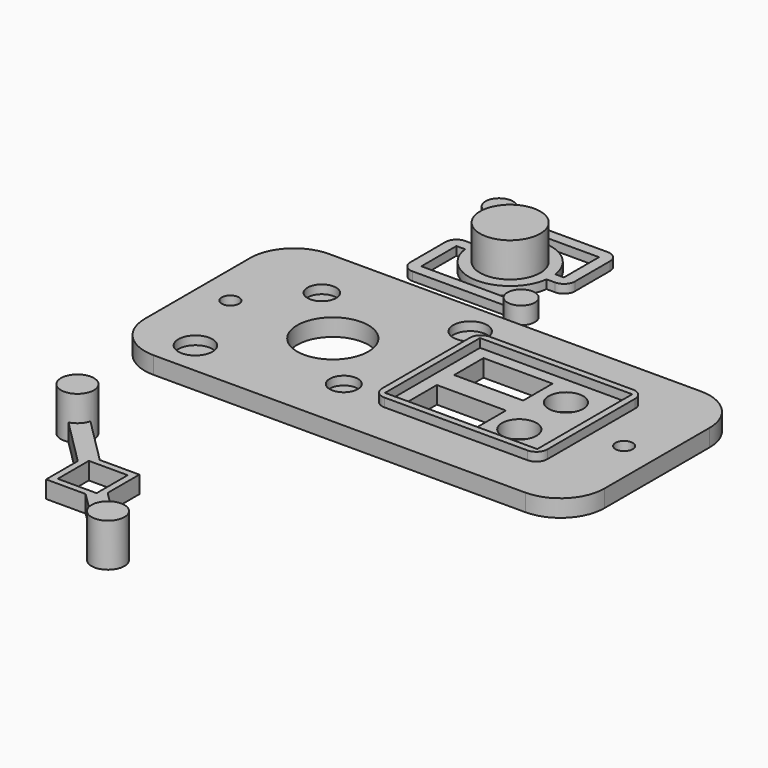
from build123d import *

# Parameters (mm, degrees)
F0_W      = 106.426
F0_H      = 50.8
F0_R      = 3.937
F0_R_2    = 3.2593015929
F0_R_3    = 2
F0_R_4    = 8.255
F0_R_5    = 3.302
F0_W_2    = 38.25
F0_H_2    = 30.5
F0_W_3    = 35.25
F0_H_3    = 27.5
F0_W_4    = 16
F0_H_4    = 8.5
F0_R_6    = 4
F1_DEPTH  = 4
F2_R      = 10.16
F3_DEPTH  = 6
F4_R      = 6.985
F4_W      = 1.27
F4_H      = 10.16
F4_H_2    = 1.27
F4_W_2    = 3
F4_H_3    = 4
F5_DEPTH  = 2
F6_DEPTH  = 10
F7_R      = 2.54
F8_DEPTH  = 4
F9_DEPTH  = 4
F10_START = 2
F10_DEPTH = 2
F11_W     = 9
F11_H     = 9
F12_DEPTH = 4
F13_R     = 2.54
F14_DEPTH = 10


# Not quite as in the source:
# - a feature names something its author has since deleted; it is built from what else it names


with BuildPart() as f1:
    # F0 (on Top) → F1 (new body)
    with BuildSketch(Plane.XY):
        with Locations((-3.608, -5.1e-06)):
            Rectangle(F0_W, F0_H)
        with Locations((-43.1534, -17.6784)):
            Circle(F0_R, mode=Mode.SUBTRACT)
        with Locations((-12.775, -12.7)):
            Circle(F0_R_2, mode=Mode.SUBTRACT)
        with Locations((-49.201, 0.0028)):
            Circle(F0_R_3, mode=Mode.SUBTRACT)
        with Locations((-25.475, 0)):
            Circle(F0_R_4, mode=Mode.SUBTRACT)
        with Locations((-38.175, 12.7)):
            Circle(F0_R_5, mode=Mode.SUBTRACT)
        with Locations((-7.7966, 17.6784)):
            Circle(F0_R, mode=Mode.SUBTRACT)
        with Locations((15.24, 0)):
            Rectangle(F0_W_2, F0_H_2, mode=Mode.SUBTRACT)
        with Locations((41.985, 0.0028)):
            Circle(F0_R_3, mode=Mode.SUBTRACT)
        with Locations((15.24, 0)):
            Rectangle(F0_W_2, F0_H_2)
        with Locations((15.24, 0)):
            Rectangle(F0_W_3, F0_H_3, mode=Mode.SUBTRACT)
        with Locations((15.24, 0)):
            Rectangle(F0_W_3, F0_H_3)
        with Locations((8.615, -6.75)):
            Rectangle(F0_W_4, F0_H_4, mode=Mode.SUBTRACT)
        with Locations((23.115, -6.75)):
            Circle(F0_R_6, mode=Mode.SUBTRACT)
        with Locations((8.615, 6.75)):
            Rectangle(F0_W_4, F0_H_4, mode=Mode.SUBTRACT)
        with Locations((23.115, 6.75)):
            Circle(F0_R_6, mode=Mode.SUBTRACT)
        with Locations((-38.175, 12.7)):
            Circle(F0_R_5)
        with Locations((-12.775, -12.7)):
            Circle(F0_R_2)
        with Locations((-7.7966, 17.6784)):
            Circle(F0_R)
        with Locations((-43.1534, -17.6784)):
            Circle(F0_R)
    extrude(amount=F1_DEPTH)

    # F2
    f2_edges = [f1.edges().sort_by_distance(p)[0] for p in [
        (-56.821, -25.400005, 2),
        (-56.821, 25.399995, 2),
        (49.605, 25.399995, 2),
        (49.605, -25.400005, 2),
    ]]
    fillet(f2_edges, radius=F2_R)

    # F0 (on Top) → F3 (join)
    with BuildSketch(Plane.XY):
        with Locations((15.24, 0)):
            Rectangle(F0_W_2, F0_H_2)
        with Locations((15.24, 0)):
            Rectangle(F0_W_3, F0_H_3, mode=Mode.SUBTRACT)
    extrude(amount=F3_DEPTH)

    # F0 (on Top) → F10 (cut)
    with BuildSketch(Plane.XY.offset(F10_START)):
        with Locations((-38.175, 12.7)):
            Circle(F0_R_5)
        with Locations((-12.775, -12.7)):
            Circle(F0_R_2)
        with Locations((-7.7966, 17.6784)):
            Circle(F0_R)
        with Locations((-43.1534, -17.6784)):
            Circle(F0_R)
    extrude(amount=F10_DEPTH, mode=Mode.SUBTRACT)

    # F13
    f13_edges = [f1.edges().sort_by_distance(p)[0] for p in [
        (-3.885, 15.25, 5),
        (34.365, 15.25, 5),
        (34.365, -15.25, 5),
        (-3.885, -15.25, 5),
    ]]
    fillet(f13_edges, radius=F13_R)


with BuildPart() as f5:
    # F4 (on Top) → F5 (new body)
    with BuildSketch(Plane.XY):
        with BuildLine():
            Line((-13.3349857867, 47.7519830668), (-12.1500321321, 47.7519830668))
            ThreePointArc((-12.1500321321, 47.7519830668), (-21.5899857867, 56.0069830668), (-31.0299394412, 47.7519830668))
            Line((-31.0299394412, 47.7519830668), (-29.8449857867, 47.7519830668))
            Line((-29.8449857867, 47.7519830668), (-29.8449857867, 45.2119830668))
            Line((-29.8449857867, 45.2119830668), (-31.0299394412, 45.2119830668))
            ThreePointArc((-31.0299394412, 45.2119830668), (-21.5899857867, 36.9569830668), (-12.1500321321, 45.2119830668))
            Line((-12.1500321321, 45.2119830668), (-13.3349857867, 45.2119830668))
            Line((-13.3349857867, 45.2119830668), (-13.3349857867, 47.7519830668))
        make_face()
        with Locations((-21.5899857867, 46.4819830668)):
            Circle(F4_R, mode=Mode.SUBTRACT)
        with BuildLine():
            ThreePointArc((-5.7149857867, 33.7819830668), (-8.241302668, 36.8900106104), (-11.799921353, 35.0519830668))
            Line((-11.799921353, 35.0519830668), (-7.6199857867, 35.0519830668))
            Line((-7.6199857867, 35.0519830668), (-7.6199857867, 32.5119830668))
            Line((-7.6199857867, 32.5119830668), (-11.799921353, 32.5119830668))
            ThreePointArc((-11.799921353, 32.5119830668), (-8.241302668, 30.6739555232), (-5.7149857867, 33.7819830668))
        make_face()
        with BuildLine():
            ThreePointArc((-31.3800502204, 60.4519830668), (-37.4649857867, 59.1819830668), (-31.3800502204, 57.9119830668))
            Line((-31.3800502204, 57.9119830668), (-34.2899857867, 57.9119830668))
            Line((-34.2899857867, 57.9119830668), (-34.2899857867, 59.1819830668))
            Line((-34.2899857867, 59.1819830668), (-34.2899857867, 60.4519830668))
            Line((-34.2899857867, 60.4519830668), (-31.3800502204, 60.4519830668))
        make_face()
        with BuildLine():
            ThreePointArc((-31.1149857867, 59.1819830668), (-31.1819582431, 59.8306661855), (-31.3800502204, 60.4519830668))
            Line((-31.3800502204, 60.4519830668), (-34.2899857867, 60.4519830668))
            Line((-34.2899857867, 60.4519830668), (-34.2899857867, 59.1819830668))
            Line((-34.2899857867, 59.1819830668), (-31.1149857867, 59.1819830668))
        make_face()
        with BuildLine():
            Line((-34.2899857867, 57.9119830668), (-31.3800502204, 57.9119830668))
            ThreePointArc((-31.3800502204, 57.9119830668), (-31.1819582431, 58.5332999481), (-31.1149857867, 59.1819830668))
            Line((-31.1149857867, 59.1819830668), (-34.2899857867, 59.1819830668))
            Line((-34.2899857867, 59.1819830668), (-34.2899857867, 57.9119830668))
        make_face()
        with BuildLine():
            Line((-31.3800502204, 57.9119830668), (-10.1599857867, 57.9119830668))
            Line((-10.1599857867, 57.9119830668), (-10.1599857867, 59.1819830668))
            Line((-10.1599857867, 59.1819830668), (-31.1149857867, 59.1819830668))
            ThreePointArc((-31.1149857867, 59.1819830668), (-31.1819582431, 58.5332999481), (-31.3800502204, 57.9119830668))
        make_face()
        with BuildLine():
            Line((-31.1149857867, 59.1819830668), (-10.1599857867, 59.1819830668))
            Line((-10.1599857867, 59.1819830668), (-10.1599857867, 60.4519830668))
            Line((-10.1599857867, 60.4519830668), (-31.3800502204, 60.4519830668))
            ThreePointArc((-31.3800502204, 60.4519830668), (-31.1819582431, 59.8306661855), (-31.1149857867, 59.1819830668))
        make_face()
        Polygon((-8.8899857867, 57.9119830668), (-8.8899857867, 47.7519830668), (-7.6199857867, 47.7519830668), (-7.6199857867, 60.4519830668), (-8.8899857867, 60.4519830668), (-8.8899857867, 59.1819830668), align=None)
        with Locations((-9.5249857867, 52.8319830668)):
            Rectangle(F4_W, F4_H)
        with Locations((-9.5249857867, 58.5469830668)):
            Rectangle(F4_W, F4_H_2)
        with Locations((-9.5249857867, 59.8169830668)):
            Rectangle(F4_W, F4_H_2)
        Polygon((-8.8899857867, 46.4819830668), (-10.1599857867, 46.4819830668), (-10.1599857867, 45.2119830668), (-7.6199857867, 45.2119830668), (-7.6199857867, 47.7519830668), (-8.8899857867, 47.7519830668), align=None)
        with Locations((-9.5249857867, 47.1169830668)):
            Rectangle(F4_W, F4_H_2)
        with BuildLine():
            ThreePointArc((-12.1500321321, 47.7519830668), (-12.0862711561, 47.1184052696), (-12.0649857867, 46.4819830668))
            Line((-12.0649857867, 46.4819830668), (-10.1599857867, 46.4819830668))
            Line((-10.1599857867, 46.4819830668), (-10.1599857867, 47.7519830668))
            Line((-10.1599857867, 47.7519830668), (-12.1500321321, 47.7519830668))
        make_face()
        with BuildLine():
            Line((-10.1599857867, 46.4819830668), (-12.0649857867, 46.4819830668))
            ThreePointArc((-12.0649857867, 46.4819830668), (-12.0862711561, 45.845560864), (-12.1500321321, 45.2119830668))
            Line((-12.1500321321, 45.2119830668), (-10.1599857867, 45.2119830668))
            Line((-10.1599857867, 45.2119830668), (-10.1599857867, 46.4819830668))
        make_face()
        with BuildLine():
            ThreePointArc((-12.1500321321, 45.2119830668), (-12.0862711561, 45.845560864), (-12.0649857867, 46.4819830668))
            ThreePointArc((-12.0649857867, 46.4819830668), (-12.0862711561, 47.1184052696), (-12.1500321321, 47.7519830668))
            Line((-12.1500321321, 47.7519830668), (-13.3349857867, 47.7519830668))
            Line((-13.3349857867, 47.7519830668), (-13.3349857867, 45.2119830668))
            Line((-13.3349857867, 45.2119830668), (-12.1500321321, 45.2119830668))
        make_face()
        with BuildLine():
            ThreePointArc((-31.1149857867, 46.4819830668), (-31.0937004173, 47.1184052696), (-31.0299394412, 47.7519830668))
            Line((-31.0299394412, 47.7519830668), (-33.0199857867, 47.7519830668))
            Line((-33.0199857867, 47.7519830668), (-33.0199857867, 46.4819830668))
            Line((-33.0199857867, 46.4819830668), (-31.1149857867, 46.4819830668))
        make_face()
        with BuildLine():
            Line((-33.0199857867, 45.2119830668), (-31.0299394412, 45.2119830668))
            ThreePointArc((-31.0299394412, 45.2119830668), (-31.0937004173, 45.845560864), (-31.1149857867, 46.4819830668))
            Line((-31.1149857867, 46.4819830668), (-33.0199857867, 46.4819830668))
            Line((-33.0199857867, 46.4819830668), (-33.0199857867, 45.2119830668))
        make_face()
        with BuildLine():
            Line((-29.8449857867, 47.7519830668), (-31.0299394412, 47.7519830668))
            ThreePointArc((-31.0299394412, 47.7519830668), (-31.0937004173, 47.1184052696), (-31.1149857867, 46.4819830668))
            ThreePointArc((-31.1149857867, 46.4819830668), (-31.0937004173, 45.845560864), (-31.0299394412, 45.2119830668))
            Line((-31.0299394412, 45.2119830668), (-29.8449857867, 45.2119830668))
            Line((-29.8449857867, 45.2119830668), (-29.8449857867, 47.7519830668))
        make_face()
        Polygon((-33.0199857867, 46.4819830668), (-33.0199857867, 47.7519830668), (-35.5599857867, 47.7519830668), (-35.5599857867, 45.2119830668), (-34.2899857867, 45.2119830668), (-34.2899857867, 46.4819830668), align=None)
        with Locations((-33.6549857867, 45.8469830668)):
            Rectangle(F4_W, F4_H_2)
        with Locations((-34.9249857867, 40.1319830668)):
            Rectangle(F4_W, F4_H)
        with Locations((-33.6549857867, 40.1319830668)):
            Rectangle(F4_W, F4_H)
        Polygon((-34.2899857867, 33.7819830668), (-34.2899857867, 35.0519830668), (-35.5599857867, 35.0519830668), (-35.5599857867, 32.5119830668), (-33.0199857867, 32.5119830668), (-33.0199857867, 33.7819830668), align=None)
        with Locations((-33.6549857867, 34.4169830668)):
            Rectangle(F4_W, F4_H_2)
        with BuildLine():
            Line((-11.799921353, 35.0519830668), (-33.0199857867, 35.0519830668))
            Line((-33.0199857867, 35.0519830668), (-33.0199857867, 33.7819830668))
            Line((-33.0199857867, 33.7819830668), (-12.0649857867, 33.7819830668))
            ThreePointArc((-12.0649857867, 33.7819830668), (-11.9980133302, 34.4306661855), (-11.799921353, 35.0519830668))
        make_face()
        with BuildLine():
            Line((-12.0649857867, 33.7819830668), (-33.0199857867, 33.7819830668))
            Line((-33.0199857867, 33.7819830668), (-33.0199857867, 32.5119830668))
            Line((-33.0199857867, 32.5119830668), (-11.799921353, 32.5119830668))
            ThreePointArc((-11.799921353, 32.5119830668), (-11.9980133302, 33.1332999481), (-12.0649857867, 33.7819830668))
        make_face()
        with BuildLine():
            Line((-7.6199857867, 35.0519830668), (-11.799921353, 35.0519830668))
            ThreePointArc((-11.799921353, 35.0519830668), (-11.9980133302, 34.4306661855), (-12.0649857867, 33.7819830668))
            ThreePointArc((-12.0649857867, 33.7819830668), (-11.9980133302, 33.1332999481), (-11.799921353, 32.5119830668))
            Line((-11.799921353, 32.5119830668), (-7.6199857867, 32.5119830668))
            Line((-7.6199857867, 32.5119830668), (-7.6199857867, 35.0519830668))
        make_face()
        with Locations((-21.5899857867, 46.4819830668)):
            Circle(F4_R)
        with Locations((-21.5899857867, 46.4819830668)):
            Rectangle(F4_W_2, F4_H_3, mode=Mode.SUBTRACT)
        with Locations((-21.5899857867, 46.4819830668)):
            Rectangle(F4_W_2, F4_H_3)
    extrude(amount=F5_DEPTH)

    # F4 (on Top) → F6 (join)
    with BuildSketch(Plane.XY):
        with Locations((-21.5899857867, 46.4819830668)):
            Circle(F4_R)
        with Locations((-21.5899857867, 46.4819830668)):
            Rectangle(F4_W_2, F4_H_3, mode=Mode.SUBTRACT)
        with Locations((-21.5899857867, 46.4819830668)):
            Rectangle(F4_W_2, F4_H_3)
    extrude(amount=F6_DEPTH)

    # F7
    f7_edges = [f5.edges().sort_by_distance(p)[0] for p in [
        (-7.619986, 60.451983, 1),
        (-7.619986, 45.211983, 1),
        (-35.559986, 32.511983, 1),
        (-35.559986, 47.751983, 1),
    ]]
    fillet(f7_edges, radius=F7_R)

    # F4 (on Top) → F8 (cut)
    with BuildSketch(Plane.XY):
        with Locations((-21.5899857867, 46.4819830668)):
            Rectangle(F4_W_2, F4_H_3)
    extrude(amount=F8_DEPTH, mode=Mode.SUBTRACT)

    # F4 (on Top) → F9 (join)
    with BuildSketch(Plane.XY):
        with BuildLine():
            ThreePointArc((-31.3800502204, 60.4519830668), (-37.4649857867, 59.1819830668), (-31.3800502204, 57.9119830668))
            Line((-31.3800502204, 57.9119830668), (-34.2899857867, 57.9119830668))
            Line((-34.2899857867, 57.9119830668), (-34.2899857867, 59.1819830668))
            Line((-34.2899857867, 59.1819830668), (-34.2899857867, 60.4519830668))
            Line((-34.2899857867, 60.4519830668), (-31.3800502204, 60.4519830668))
        make_face()
        with BuildLine():
            ThreePointArc((-31.1149857867, 59.1819830668), (-31.1819582431, 59.8306661855), (-31.3800502204, 60.4519830668))
            Line((-31.3800502204, 60.4519830668), (-34.2899857867, 60.4519830668))
            Line((-34.2899857867, 60.4519830668), (-34.2899857867, 59.1819830668))
            Line((-34.2899857867, 59.1819830668), (-31.1149857867, 59.1819830668))
        make_face()
        with BuildLine():
            Line((-34.2899857867, 57.9119830668), (-31.3800502204, 57.9119830668))
            ThreePointArc((-31.3800502204, 57.9119830668), (-31.1819582431, 58.5332999481), (-31.1149857867, 59.1819830668))
            Line((-31.1149857867, 59.1819830668), (-34.2899857867, 59.1819830668))
            Line((-34.2899857867, 59.1819830668), (-34.2899857867, 57.9119830668))
        make_face()
        with BuildLine():
            ThreePointArc((-5.7149857867, 33.7819830668), (-8.241302668, 36.8900106104), (-11.799921353, 35.0519830668))
            Line((-11.799921353, 35.0519830668), (-7.6199857867, 35.0519830668))
            Line((-7.6199857867, 35.0519830668), (-7.6199857867, 32.5119830668))
            Line((-7.6199857867, 32.5119830668), (-11.799921353, 32.5119830668))
            ThreePointArc((-11.799921353, 32.5119830668), (-8.241302668, 30.6739555232), (-5.7149857867, 33.7819830668))
        make_face()
        with BuildLine():
            Line((-7.6199857867, 35.0519830668), (-11.799921353, 35.0519830668))
            ThreePointArc((-11.799921353, 35.0519830668), (-11.9980133302, 34.4306661855), (-12.0649857867, 33.7819830668))
            ThreePointArc((-12.0649857867, 33.7819830668), (-11.9980133302, 33.1332999481), (-11.799921353, 32.5119830668))
            Line((-11.799921353, 32.5119830668), (-7.6199857867, 32.5119830668))
            Line((-7.6199857867, 32.5119830668), (-7.6199857867, 35.0519830668))
        make_face()
    extrude(amount=F9_DEPTH)


with BuildPart() as f12:
    # F11 (on Top) → F12 (new body)
    with BuildSketch(Plane.XY):
        with BuildLine():
            ThreePointArc((-42.2705026911, -55.5329295336), (-41.2924403918, -55.152540039), (-40.4552561211, -54.5197489789))
            ThreePointArc((-40.4552561211, -54.5197489789), (-39.822465061, -53.6825647082), (-39.4420755664, -52.7045024089))
            ThreePointArc((-39.4420755664, -52.7045024089), (-39.36510578, -52.2680799524), (-39.3393329574, -51.8256721426))
            ThreePointArc((-39.3393329574, -51.8256721426), (-46.1380152184, -49.4626490063), (-42.2705026911, -55.5329295336))
        make_face()
        with BuildLine():
            Line((-40.4552561211, -54.5197489789), (-31.475, -63.5000051))
            Line((-31.475, -63.5000051), (-28.6465728753, -63.5000051))
            Line((-28.6465728753, -63.5000051), (-39.4420755664, -52.7045024089))
            ThreePointArc((-39.4420755664, -52.7045024089), (-39.822465061, -53.6825647082), (-40.4552561211, -54.5197489789))
        make_face()
        with BuildLine():
            Line((-31.475, -66.3284322247), (-31.475, -63.5000051))
            Line((-31.475, -63.5000051), (-40.4552561211, -54.5197489789))
            ThreePointArc((-40.4552561211, -54.5197489789), (-41.2924403918, -55.152540039), (-42.2705026911, -55.5329295336))
            Line((-42.2705026911, -55.5329295336), (-31.475, -66.3284322247))
        make_face()
        Polygon((-28.6465728753, -63.5000051), (-31.475, -63.5000051), (-31.475, -66.3284322247), (-31.475, -75.5000051), (-22.3034271247, -75.5000051), (-19.475, -75.5000051), (-19.475, -72.6715779753), (-19.475, -63.5000051), align=None)
        with Locations((-25.475, -69.5000051)):
            Rectangle(F11_W, F11_H, mode=Mode.SUBTRACT)
        with BuildLine():
            Line((-8.6794973089, -83.4670806664), (-19.475, -72.6715779753))
            Line((-19.475, -72.6715779753), (-19.475, -75.5000051))
            Line((-19.475, -75.5000051), (-10.4947438789, -84.4802612211))
            ThreePointArc((-10.4947438789, -84.4802612211), (-9.6575596082, -83.847470161), (-8.6794973089, -83.4670806664))
        make_face()
        with BuildLine():
            Line((-19.475, -75.5000051), (-22.3034271247, -75.5000051))
            Line((-22.3034271247, -75.5000051), (-11.5079244336, -86.2955077911))
            ThreePointArc((-11.5079244336, -86.2955077911), (-11.127534939, -85.3174454918), (-10.4947438789, -84.4802612211))
            Line((-10.4947438789, -84.4802612211), (-19.475, -75.5000051))
        make_face()
        with BuildLine():
            ThreePointArc((-3.9906670426, -87.1743380574), (-5.4376439063, -84.1856557964), (-8.6794973089, -83.4670806664))
            ThreePointArc((-8.6794973089, -83.4670806664), (-9.6575596082, -83.847470161), (-10.4947438789, -84.4802612211))
            ThreePointArc((-10.4947438789, -84.4802612211), (-11.127534939, -85.3174454918), (-11.5079244336, -86.2955077911))
            ThreePointArc((-11.5079244336, -86.2955077911), (-8.2430748524, -90.9585652347), (-3.9906670426, -87.1743380574))
        make_face()
    extrude(amount=F12_DEPTH)

    # F11 (on Top) → F14 (join)
    with BuildSketch(Plane.XY):
        with BuildLine():
            ThreePointArc((-42.2705026911, -55.5329295336), (-41.2924403918, -55.152540039), (-40.4552561211, -54.5197489789))
            ThreePointArc((-40.4552561211, -54.5197489789), (-39.822465061, -53.6825647082), (-39.4420755664, -52.7045024089))
            ThreePointArc((-39.4420755664, -52.7045024089), (-39.36510578, -52.2680799524), (-39.3393329574, -51.8256721426))
            ThreePointArc((-39.3393329574, -51.8256721426), (-46.1380152184, -49.4626490063), (-42.2705026911, -55.5329295336))
        make_face()
        with BuildLine():
            ThreePointArc((-3.9906670426, -87.1743380574), (-5.4376439063, -84.1856557964), (-8.6794973089, -83.4670806664))
            ThreePointArc((-8.6794973089, -83.4670806664), (-9.6575596082, -83.847470161), (-10.4947438789, -84.4802612211))
            ThreePointArc((-10.4947438789, -84.4802612211), (-11.127534939, -85.3174454918), (-11.5079244336, -86.2955077911))
            ThreePointArc((-11.5079244336, -86.2955077911), (-8.2430748524, -90.9585652347), (-3.9906670426, -87.1743380574))
        make_face()
    extrude(amount=F14_DEPTH)


solid = Compound([f1.part, f5.part, f12.part])
